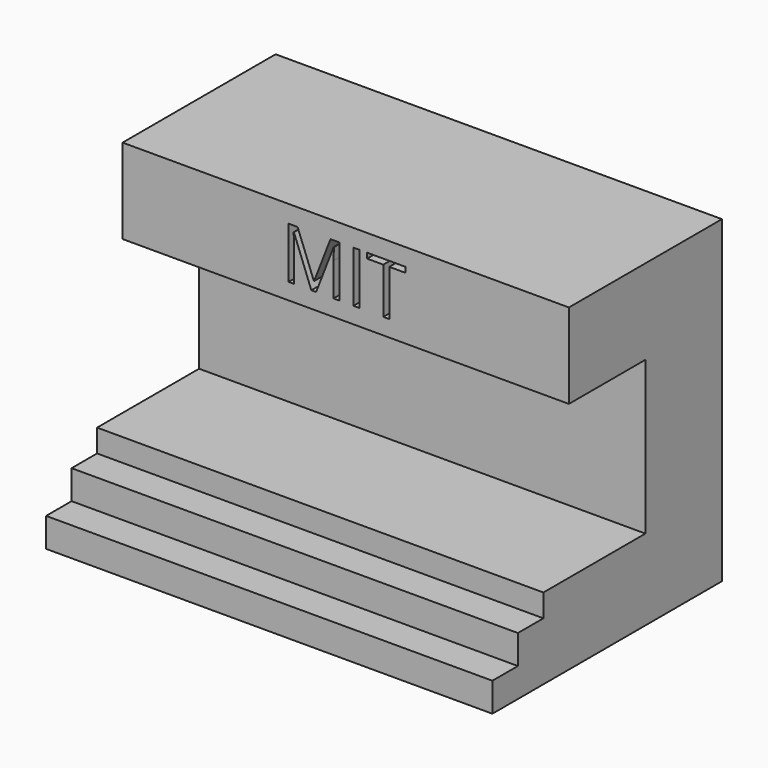
from build123d import *

# Parameters (mm, degrees)
F0_W          = 88.9
F0_H          = 38.1
F1_DEPTH      = 63.5
F2_W          = 88.9
F2_H          = 30.48
F3_DEPTH      = 19.05
F4_W          = 88.9
F4_H          = 4.5306356624
F5_DEPTH      = 6.35
F6_W          = 88.9
F6_H          = 5.7859825902
F7_DEPTH      = 12.7
F8_W          = 88.9
F8_H          = 5.7859825902
F9_DEPTH      = 19.05
F10_TEXT_SIZE = 14.30651173
F11_DEPTH     = 5.08


# Not quite as in the source:
# - Text() gives the source's letters only with a copy of the font that has no kerning and outlines rounded to 1/6400 em; it was checked with that copy


with BuildPart() as f1:
    # F0 (on Top) → F1 (new body)
    with BuildSketch(Plane.XY):
        with Locations((-1.113217324, -0.6447832179)):
            Rectangle(F0_W, F0_H)
    extrude(amount=F1_DEPTH)

    # F2 (on face) → F3 (cut)
    with BuildSketch(Plane.XZ.offset(19.6947832179)):
        with Locations((-1.113217324, 31.3426008427)):
            Rectangle(F2_W, F2_H)
    extrude(amount=-F3_DEPTH, mode=Mode.SUBTRACT)

    # F4 (on face) → F5 (join)
    with BuildSketch(Plane.XZ.offset(19.6947832179)):
        with Locations((-1.113217324, 13.8372830115)):
            Rectangle(F4_W, F4_H)
    extrude(amount=F5_DEPTH)

    # F6 (on face) → F7 (join)
    with BuildSketch(Plane.XZ.offset(19.6947832179)):
        with Locations((-1.113217324, 8.6789738853)):
            Rectangle(F6_W, F6_H)
    extrude(amount=F7_DEPTH)

    # F8 (on face) → F9 (join)
    with BuildSketch(Plane.XZ.offset(19.6947832179)):
        with Locations((-1.113217324, 2.8929912951)):
            Rectangle(F8_W, F8_H)
    extrude(amount=F9_DEPTH)

    # F10 (on face) → F11 (cut)
    with BuildSketch(Plane.XZ.offset(19.6947832179)):
        with Locations((-13.893954223, 49.8265884817)):
            Text('MIT', F10_TEXT_SIZE, font='Open Sans', text_align=(TextAlign.LEFT, TextAlign.BOTTOM))
    extrude(amount=-F11_DEPTH, mode=Mode.SUBTRACT)


solid = f1.part
